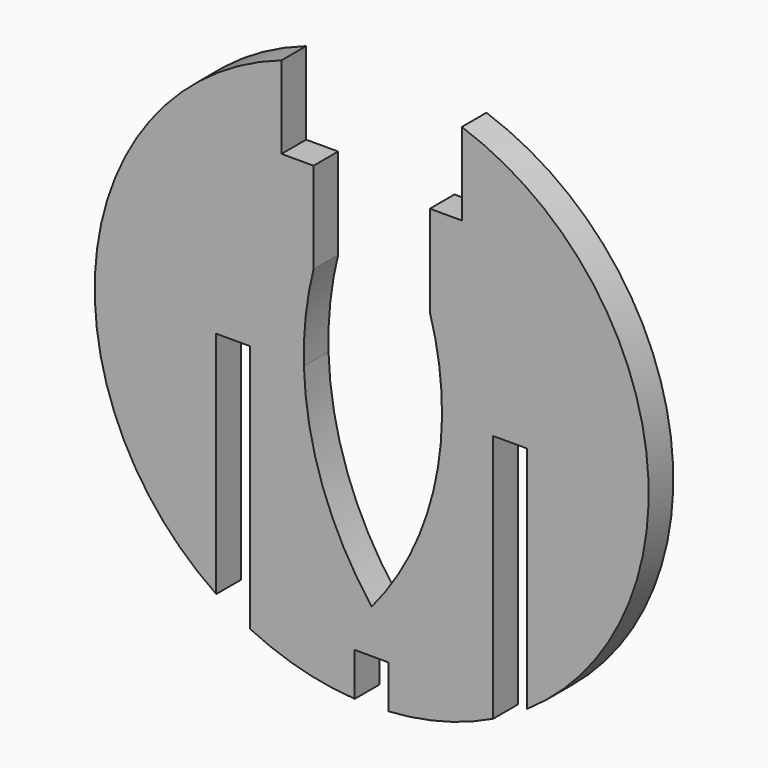
from build123d import *

# Parameters (mm, degrees)
F0_R     = 28.575
F1_DEPTH = 3.175
F3_DEPTH = 3.176


# Not quite as in the source:
# - a length typed as a fraction of an inch, garbled in the dataset ("3 / 203.2 mm" for 3/8 in), is restored


with BuildPart() as f1:
    # F0 (on Front) → F1 (new body)
    with BuildSketch(Plane.XZ):
        Circle(F0_R)
    extrude(amount=F1_DEPTH)

    # F2 (on face) → F3 (cut, through all)
    with BuildSketch(Plane.XZ.offset(3.175)):
        with BuildLine():
            Line((7.2536082684, 0), (0, 0))
            Line((0, 0), (0, -19.575))
            ThreePointArc((0, -19.575), (5.3192801015, -10.4146549257), (7.2536082684, 0))
        make_face()
        with BuildLine():
            Line((0, -19.575), (0, 0))
            Line((0, 0), (-6.9936556862, 0))
            ThreePointArc((-6.9936556862, 0), (-5.0483188999, -10.341808774), (0, -19.575))
        make_face()
        with BuildLine():
            ThreePointArc((-6, 9.1323722154), (-6.8103344804, 4.6002974695), (-6.9936556862, 0))
            Line((-6.9936556862, 0), (0, 0))
            Line((0, 0), (7.2536082684, 0))
            ThreePointArc((7.2536082684, 0), (6.9672213091, 4.6129154541), (6, 9.1323722154))
            Line((6, 9.1323722154), (6, 18.5192639611))
            Line((6, 18.5192639611), (9.3, 18.5192639611))
            Line((9.3, 18.5192639611), (9.3, 27.0192639611))
            ThreePointArc((9.3, 27.0192639611), (0, 28.575), (-9.3, 27.0192639611))
            Line((-9.3, 27.0192639611), (-9.3, 18.5192639611))
            Line((-9.3, 18.5192639611), (-6, 18.5192639611))
            Line((-6, 18.5192639611), (-6, 9.1323722154))
        make_face()
        with BuildLine():
            ThreePointArc((-16.0375, -23.650142045), (-14.3234197578, -24.7259028438), (-12.5375, -25.6776501797))
            Line((-12.5375, -25.6776501797), (-12.5375, 0))
            Line((-12.5375, 0), (-16.0375, 0))
            Line((-16.0375, 0), (-16.0375, -23.650142045))
        make_face()
        with BuildLine():
            Line((-1.75, -24.075), (-1.75, -28.5213626077))
            ThreePointArc((-1.75, -28.5213626077), (-0.8754108992, -28.5615875042), (0, -28.575))
            Line((0, -28.575), (0, -24.075))
            Line((0, -24.075), (-1.75, -24.075))
        make_face()
        with BuildLine():
            Line((0, -24.075), (0, -28.575))
            ThreePointArc((0, -28.575), (0.8754108992, -28.5615875042), (1.75, -28.5213626077))
            Line((1.75, -28.5213626077), (1.75, -24.075))
            Line((1.75, -24.075), (0, -24.075))
        make_face()
        with BuildLine():
            Line((12.5375, 0), (12.5375, -25.6776501797))
            ThreePointArc((12.5375, -25.6776501797), (14.3234197578, -24.7259028438), (16.0375, -23.650142045))
            Line((16.0375, -23.650142045), (16.0375, 0))
            Line((16.0375, 0), (12.5375, 0))
        make_face()
    extrude(amount=-F3_DEPTH, mode=Mode.SUBTRACT)


solid = f1.part
